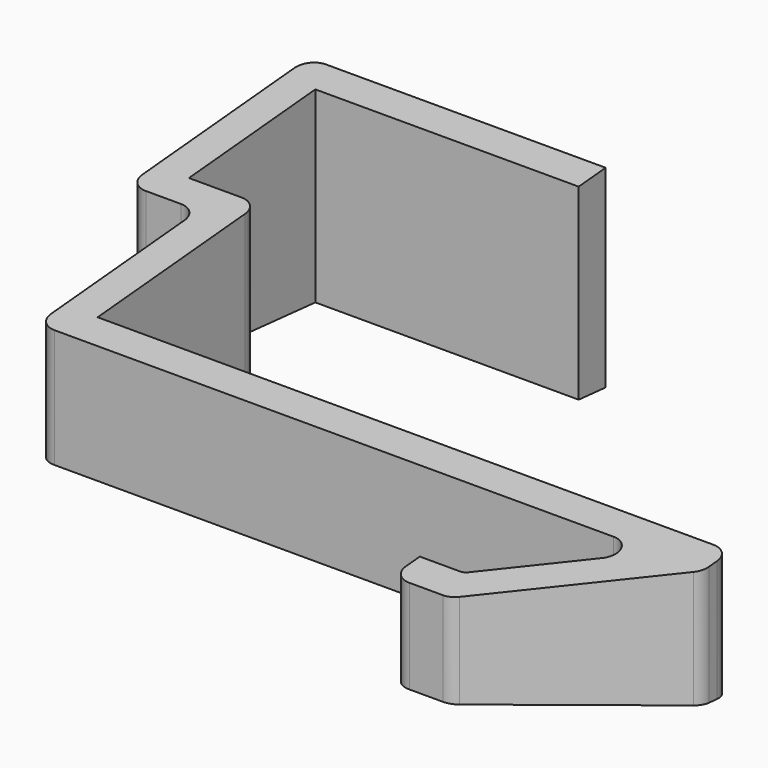
from build123d import *

# Parameters (mm, degrees)
F1_DEPTH = 30
F5_REACH = 130.7668048394
F6_DEPTH = 30
F8_R     = 2


# Not quite as in the source:
# - two fillets or chamfers of one size are made in one step


with BuildPart() as f1:
    # F0 (on Top) → F1 (new body, symmetric)
    with BuildSketch(Plane.XY):
        with BuildLine():
            Line((-2.159999702, 23), (-10.159999702, 23))
            Line((-10.159999702, 23), (-10.159999702, 41))
            Line((-10.159999702, 41), (19.840000298, 41))
            Line((19.840000298, 41), (19.840000298, 44.84))
            Line((19.840000298, 44.84), (-13.999999702, 44.84))
            Line((-13.999999702, 44.84), (-13.999999702, 19.16))
            Line((-13.999999702, 19.16), (-5.999999702, 19.16))
            Line((-5.999999702, 19.16), (-5.999999702, -3.84))
            Line((-5.999999702, -3.84), (64.5031457505, -3.84))
            Line((64.5031457505, -3.84), (52.6360389693, -15.7071067812))
            ThreePointArc((52.6360389693, -15.7071067812), (52.3116156205, -15.9238795325), (51.9289321881, -16))
            Line((51.9289321881, -16), (47.3431457505, -16))
            Line((47.3431457505, -16), (47.3431457505, -20))
            Line((47.3431457505, -20), (54, -20))
            Line((54, -20), (70, -4))
            Line((70, -4), (70, 0))
            Line((70, 0), (-2.159999702, 0))
            Line((-2.159999702, 0), (-2.159999702, 23))
        make_face()
    extrude(amount=F1_DEPTH, both=True)

    f5_end = Plane(origin=(0, -0.6162060448, 7.0432673219), x_dir=(0, 0.9961946981, 0.0871557427), z_dir=(0, -0.0871557427, 0.9961946981))
    # F1_face2 (on face) → F5 (cut, up to a plane its end follows)
    with BuildSketch(Plane(origin=(19.935386065, 10.6416249654, 30), x_dir=(1, 0, 0), z_dir=(0, 0, 1))):
        with BuildLine():
            Line((-22.095385767, -10.6416249654), (-22.095385767, 12.3583750346))
            Line((-22.095385767, 12.3583750346), (-30.095385767, 12.3583750346))
            Line((-30.095385767, 12.3583750346), (-30.095385767, 30.3583750346))
            Line((-30.095385767, 30.3583750346), (-0.095385767, 30.3583750346))
            Line((-0.095385767, 30.3583750346), (-0.095385767, 34.1983750346))
            Line((-0.095385767, 34.1983750346), (-33.935385767, 34.1983750346))
            Line((-33.935385767, 34.1983750346), (-33.935385767, 8.5183750346))
            Line((-33.935385767, 8.5183750346), (-25.935385767, 8.5183750346))
            Line((-25.935385767, 8.5183750346), (-25.935385767, -14.4816249654))
            Line((-25.935385767, -14.4816249654), (44.5677596855, -14.4816249654))
            Line((44.5677596855, -14.4816249654), (32.7006529043, -26.3487317465))
            ThreePointArc((32.7006529043, -26.3487317465), (32.3762295555, -26.5655044979), (31.9935461231, -26.6416249654))
            Line((31.9935461231, -26.6416249654), (27.4077596855, -26.6416249654))
            Line((27.4077596855, -26.6416249654), (27.4077596855, -30.6416249654))
            Line((27.4077596855, -30.6416249654), (34.064613935, -30.6416249654))
            Line((34.064613935, -30.6416249654), (50.064613935, -14.6416249654))
            Line((50.064613935, -14.6416249654), (50.064613935, -10.6416249654))
            Line((50.064613935, -10.6416249654), (-22.095385767, -10.6416249654))
        make_face()
    f5_long = extrude(amount=-F5_REACH, mode=Mode.PRIVATE)
    add(split(f5_long, bisect_by=f5_end, keep=Keep.TOP, mode=Mode.PRIVATE), mode=Mode.SUBTRACT)

    # F6 (cut, through all): a face of the model
    f6_faces = [f1.faces().sort_by_distance(p)[0] for p in [
        (-3.2211418013, 11.5, -30),
    ]]
    extrude(f6_faces, amount=-F6_DEPTH, mode=Mode.SUBTRACT)

    # F7: F1 across plane


with BuildPart() as f1_1:
    add(f1.part)
    add(f1.part.mirror(Plane.XY))

    # F8
    f8_edges = [f1_1.edges().sort_by_distance(p)[0] for p in [
        (70, 0, 0),
        (70, -4, 0),
        (54, -20, 0),
        (47.343146, -20, 0),
        (-2.16, 23, 0),
        (-14, 44.84, 0),
        (-14, 19.16, 0),
        (-6, 19.16, 0),
        (-6, -3.84, 0),
        (64.503146, -3.84, 0),
    ]]
    fillet(f8_edges, radius=F8_R)


solid = f1_1.part
